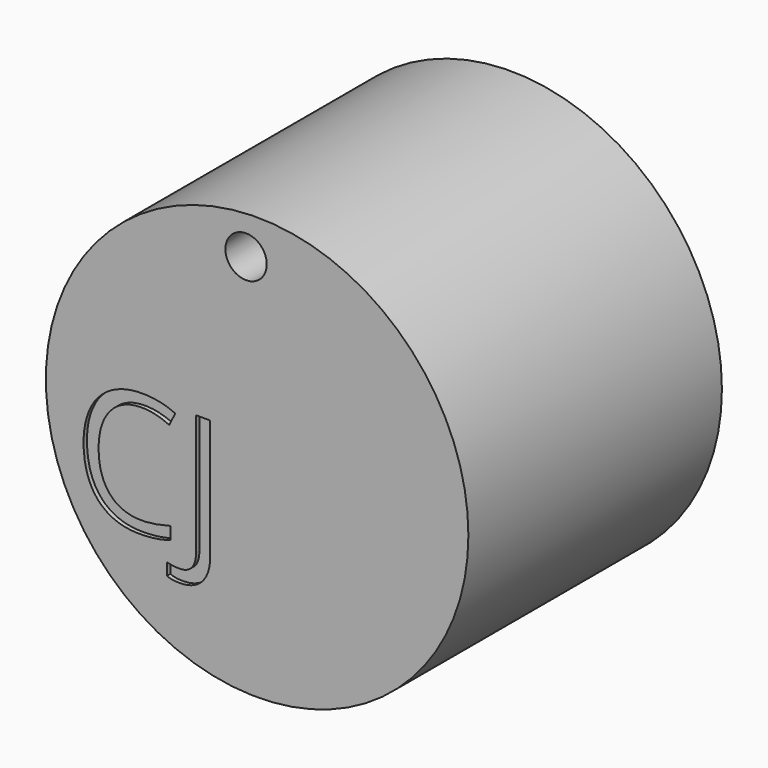
from build123d import *

# Parameters (mm, degrees)
F0_R         = 12.7
F1_DEPTH     = 19.05
F2_TEXT_SIZE = 10.2000717103
F3_DEPTH     = 0.254
F4_R         = 1.2427399659
F5_DEPTH     = 19.051
F6_TEXT_SIZE = 3.6823506569
F7_DEPTH     = 0.127
F8_TEXT_SIZE = 3.4508305472
F9_DEPTH     = 0.127


# Not quite as in the source:
# - Text() gives the source's letters only with a copy of the font that has no kerning and outlines rounded to 1/6400 em; it was checked with that copy


with BuildPart() as f1:
    # F0 (on Front) → F1 (new body)
    with BuildSketch(Plane.XZ):
        with Locations((0.6611607197, 0)):
            Circle(F0_R)
    extrude(amount=F1_DEPTH)

    # F2 (on face) → F3 (cut)
    with BuildSketch(Plane.XZ.offset(19.05)):
        with Locations((-10.3932331531, -6.2522296906)):
            Text('CJ', F2_TEXT_SIZE, font='Open Sans', text_align=(TextAlign.LEFT, TextAlign.BOTTOM))
    extrude(amount=-F3_DEPTH, mode=Mode.SUBTRACT)

    # F4 (on face) → F5 (cut, through all)
    with BuildSketch(Plane.XZ.offset(19.05)):
        with Locations((-0.0027612196, 10.3953736052)):
            Circle(F4_R)
    extrude(amount=-F5_DEPTH, mode=Mode.SUBTRACT)

    # F6 (on face) → F7 (cut, symmetric)
    with BuildSketch(Plane(origin=(0, 0, 0), x_dir=(-1, 0, 0), z_dir=(0, 1, 0))):
        with Locations((-9.4808079448, 1.8269762517)):
            Text('Wrestling', F6_TEXT_SIZE, font='Open Sans', font_style=FontStyle.BOLD, text_align=(TextAlign.LEFT, TextAlign.BOTTOM))
    extrude(amount=F7_DEPTH, both=True, mode=Mode.SUBTRACT)

    # F8 (on face) → F9 (cut, symmetric)
    with BuildSketch(Plane(origin=(0, 0, 0), x_dir=(-1, 0, 0), z_dir=(0, 1, 0))):
        with Locations((-5.36567863, -3.5260976642)):
            Text('RMHS', F8_TEXT_SIZE, font='Open Sans', font_style=FontStyle.BOLD, text_align=(TextAlign.LEFT, TextAlign.BOTTOM))
    extrude(amount=F9_DEPTH, both=True, mode=Mode.SUBTRACT)


solid = f1.part
